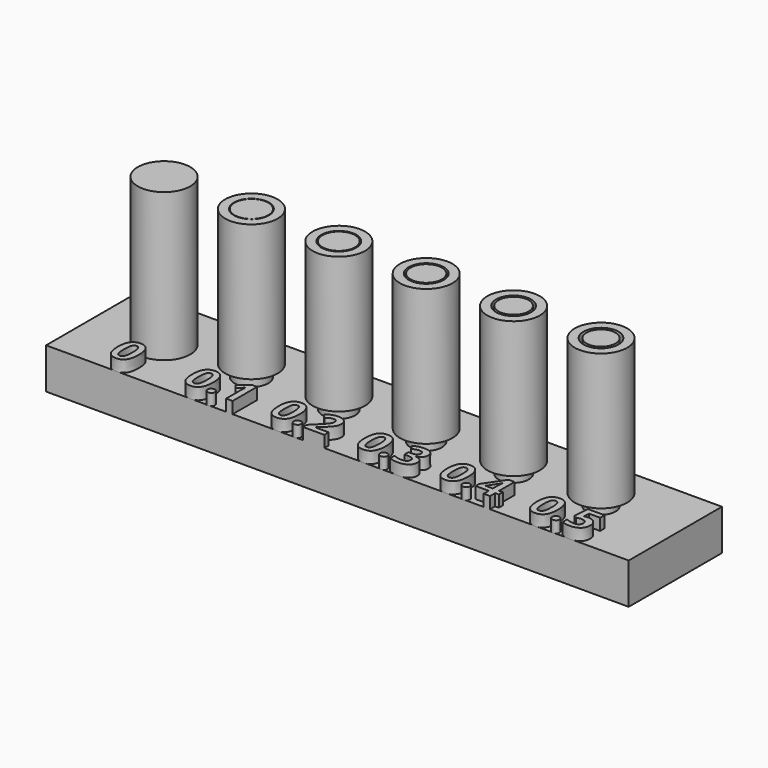
from build123d import *

# Parameters (mm, degrees)
F0_W         = 100
F0_H         = 20
F1_DEPTH     = 7
F2_R         = 4.5
F2_R_2       = 3
F2_R_3       = 2.5
F2_R_4       = 2.6
F2_R_5       = 2.7
F2_R_6       = 2.8
F2_R_7       = 2.9
F3_DEPTH     = 25.4
F4_TEXT_SIZE = 7.3535933625
F5_DEPTH     = 2
F6_R         = 4.7188672927
F6_R_2       = 2.9481003395
F6_R_3       = 4.9099464488
F6_R_4       = 2.9311630298
F6_R_5       = 4.7802242436
F6_R_6       = 2.88827331
F6_R_7       = 4.7210787776
F6_R_8       = 2.787771364
F6_R_9       = 4.7407748992
F6_R_10      = 2.7686331559
F7_DEPTH     = 2


# Not quite as in the source:
# - Text() gives the source's letters only with a copy of the font that has no kerning and outlines rounded to 1/6400 em; it was checked with that copy


with BuildPart() as f1:
    # F0 (on Top) → F1 (new body)
    with BuildSketch(Plane.XY):
        Rectangle(F0_W, F0_H)
    extrude(amount=F1_DEPTH)

    # F2 (on face) → F3 (join)
    with BuildSketch(Plane.XY.offset(7)):
        with Locations((-37.7527128436, 0)):
            Circle(F2_R)
        with Locations((-37.7527128436, 0)):
            Circle(F2_R_2, mode=Mode.SUBTRACT)
        with Locations((-22.7527128436, 0)):
            Circle(F2_R)
        with Locations((-22.7527128436, 0)):
            Circle(F2_R_2, mode=Mode.SUBTRACT)
        with Locations((-7.7527128436, 0)):
            Circle(F2_R)
        with Locations((-7.7527128436, 0)):
            Circle(F2_R_2, mode=Mode.SUBTRACT)
        with Locations((7.2472871564, 0)):
            Circle(F2_R)
        with Locations((7.2472871564, 0)):
            Circle(F2_R_2, mode=Mode.SUBTRACT)
        with Locations((22.2472871564, 0)):
            Circle(F2_R)
        with Locations((22.2472871564, 0)):
            Circle(F2_R_2, mode=Mode.SUBTRACT)
        with Locations((37.2472871564, 0)):
            Circle(F2_R)
        with Locations((37.2472871564, 0)):
            Circle(F2_R_2, mode=Mode.SUBTRACT)
        with Locations((37.2472871564, 0)):
            Circle(F2_R_3)
        with Locations((22.2472871564, 0)):
            Circle(F2_R_4)
        with Locations((7.2472871564, 0)):
            Circle(F2_R_5)
        with Locations((-7.7527128436, 0)):
            Circle(F2_R_6)
        with Locations((-22.7527128436, 0)):
            Circle(F2_R_7)
        with Locations((-37.7527128436, 0)):
            Circle(F2_R_2)
    extrude(amount=F3_DEPTH)

    # F4 (on face) → F5 (join)
    with BuildSketch(Plane.XY.offset(7)):
        with Locations((-40.1029326022, -10)):
            Text('0', F4_TEXT_SIZE, font='Open Sans', font_style=FontStyle.BOLD, text_align=(TextAlign.LEFT, TextAlign.BOTTOM))
        with Locations((-27.3139830679, -10)):
            Text('0.1', F4_TEXT_SIZE, font='Open Sans', font_style=FontStyle.BOLD, text_align=(TextAlign.LEFT, TextAlign.BOTTOM))
        with Locations((-12.5067550689, -10)):
            Text('0.2', F4_TEXT_SIZE, font='Open Sans', font_style=FontStyle.BOLD, text_align=(TextAlign.LEFT, TextAlign.BOTTOM))
        with Locations((2.3177135736, -10)):
            Text('0.3', F4_TEXT_SIZE, font='Open Sans', font_style=FontStyle.BOLD, text_align=(TextAlign.LEFT, TextAlign.BOTTOM))
        with Locations((16.4550673217, -10)):
            Text('0.4', F4_TEXT_SIZE, font='Open Sans', font_style=FontStyle.BOLD, text_align=(TextAlign.LEFT, TextAlign.BOTTOM))
        with Locations((31.8480208516, -10)):
            Text('0.5', F4_TEXT_SIZE, font='Open Sans', font_style=FontStyle.BOLD, text_align=(TextAlign.LEFT, TextAlign.BOTTOM))
    extrude(amount=F5_DEPTH)

    # F6 (on face) → F7 (cut)
    with BuildSketch(Plane.XY.offset(7)):
        with Locations((-22.7527128436, 0)):
            Circle(F6_R)
        with Locations((-22.7527128436, 0)):
            Circle(F6_R_2, mode=Mode.SUBTRACT)
        with Locations((-7.7527128436, 0)):
            Circle(F6_R_3)
        with Locations((-7.7527128436, 0)):
            Circle(F6_R_4, mode=Mode.SUBTRACT)
        with Locations((7.2472871564, 0)):
            Circle(F6_R_5)
        with Locations((7.2472871564, 0)):
            Circle(F6_R_6, mode=Mode.SUBTRACT)
        with Locations((22.2472871564, 0)):
            Circle(F6_R_7)
        with Locations((22.2472871564, 0)):
            Circle(F6_R_8, mode=Mode.SUBTRACT)
        with Locations((37.2472871564, 0)):
            Circle(F6_R_9)
        with Locations((37.2472871564, 0)):
            Circle(F6_R_10, mode=Mode.SUBTRACT)
    extrude(amount=F7_DEPTH, mode=Mode.SUBTRACT)


solid = f1.part
